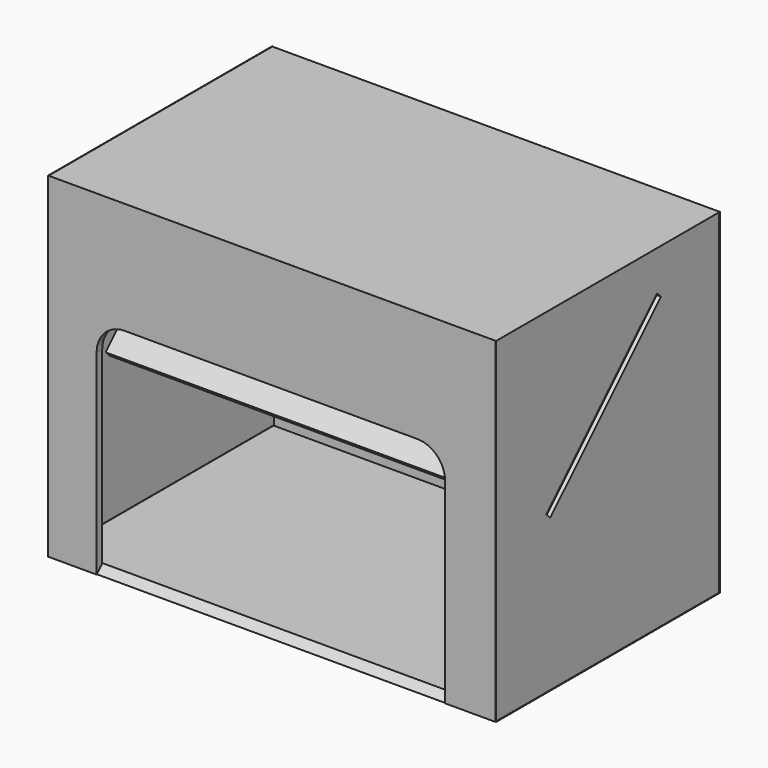
from build123d import *

# Parameters (mm, degrees)
F0_W           = 406.4
F0_H           = 254
F1_DEPTH       = 6.35
F2_SIZE        = 6.34999
F3_W           = 406.4
F3_H           = 304.8
F4_DEPTH       = 6.35
F5_SIZE        = 6.34999
F7_D           = 44.45
F7_CBORE_D     = 50.8
F7_CBORE_DEPTH = 3.175
F8_W           = 192.7503757179
F8_H           = 6.3895136118
F9_DEPTH       = 355.6
F10_ANGLE      = -45
F13_SIZE       = 2.54
F17_W          = 254
F17_H          = 304.8
F18_DEPTH      = 6.35
F20_SIZE       = 6.34999
F22_DEPTH      = 400.05
F24_DEPTH      = 3.175
F25_W          = 349.25
F25_H          = 127
F26_DEPTH      = 3.175
F29_DEPTH      = 25.4
F30_W          = 406.4
F30_H          = 304.8
F31_DEPTH      = 6.35
F32_SIZE       = 6.34999
F35_DEPTH      = 6.35
F39_W          = 406.4
F39_H          = 254
F40_DEPTH      = 6.35
F43_W          = 406.4
F43_H          = 254
F44_DEPTH      = 6.35
F46_SIZE       = 6.34999


# Not quite as in the source:
# - a fillet or chamfer is up to 0.001 mm smaller than in the source, because OpenCascade refuses the exact size


with BuildPart() as f1:
    # F0 (on Top) → F1 (new body)
    with BuildSketch(Plane.XY):
        with Locations((4.1009858251, 30.9985745514)):
            Rectangle(F0_W, F0_H)
    extrude(amount=F1_DEPTH)

    # F2 (size 6.35 in the source; OpenCascade refuses exactly that, so slightly less here)
    f2_edges = [f1.edges().sort_by_distance(p)[0] for p in [
        (-199.099014, 30.998575, 6.35),
        (4.100986, 157.998575, 6.35),
        (4.100986, -96.001425, 6.35),
        (207.300986, 30.998575, 6.35),
    ]]
    chamfer(f2_edges, length=F2_SIZE)


with BuildPart() as f4:
    # F3 (on Front) → F4 (new body)
    with BuildSketch(Plane.XZ):
        with Locations((84.3813158572, 276.6985837005)):
            Rectangle(F3_W, F3_H)
    extrude(amount=F4_DEPTH)

    # F5 (size 6.35 in the source; OpenCascade refuses exactly that, so slightly less here)
    f5_edges = [f4.edges().sort_by_distance(p)[0] for p in [
        (84.381316, -6.35, 124.298584),
        (287.581316, -6.35, 276.698584),
        (-118.818684, -6.35, 276.698584),
        (84.381316, -6.35, 429.098584),
    ]]
    chamfer(f5_edges, length=F5_SIZE)

    # F7 (through all)
    with Locations(Plane(origin=(0, 0, 0), x_dir=(-1, 0, 0), z_dir=(0, 1, 0))):
        with Locations((-84.3885657899, 327.5033756889)):
            CounterBoreHole(F7_D / 2, F7_CBORE_D / 2, F7_CBORE_DEPTH)


with BuildPart() as f9:
    # F8 (on Right) → F9 (new body)
    with BuildSketch(Plane.YZ):
        with Locations((-139.9461273104, 135.7569471002)):
            Rectangle(F8_W, F8_H)
    extrude(amount=F9_DEPTH)


with BuildPart() as f9_1:
    # F10: moved
    add(f9.part.rotate(Axis((177.8, -236.3213151693, 132.5621902943), (-1, 0, 0)), F10_ANGLE))


with BuildPart() as f9_2:
    # F11: moved
    add(f9_1.part.moved(Location((-101.6, 0, 0))))


with BuildPart() as f9_3:
    # F12: moved
    add(f9_2.part.moved(Location((0, 71.8420489686, -71.8420489686))))

    # F13
    f13_edges = [f9_3.edges().sort_by_distance(p)[0] for p in [
        (254, -96.331717, 128.86769),
        (254, -100.849786, 133.385759),
    ]]
    chamfer(f13_edges, length=F13_SIZE)


with BuildPart() as f4_1:
    # F14: moved
    add(f4.part.moved(Location((0, 152.4, -127))))


with BuildPart() as f1_1:
    # F15: moved
    add(f1.part.moved(Location((0, -5.08, -2.54))))


with BuildPart() as f4_2:
    # F16: moved
    add(f4_1.part.moved(Location((-80.01, 0, 0))))


with BuildPart() as f18:
    # F17 (on Right) → F18 (new body)
    with BuildSketch(Plane.YZ):
        with Locations((26.0427181125, 152.4)):
            Rectangle(F17_W, F17_H)
    extrude(amount=F18_DEPTH)


with BuildPart() as f18_1:
    # F19: moved
    add(f18.part.moved(Location((-199.39, 0, -2.54))))

    # F20 (size 6.35 in the source; OpenCascade refuses exactly that, so slightly less here)
    f20_edges = [f18_1.edges().sort_by_distance(p)[0] for p in [
        (-193.04, 26.042718, -2.54),
        (-193.04, -100.957282, 149.86),
        (-193.04, 153.042718, 149.86),
        (-193.04, 26.042718, 302.26),
    ]]
    chamfer(f20_edges, length=F20_SIZE)

    # F23 (on face) → F24 (cut)
    with BuildSketch(Plane.YZ.offset(-193.04)):
        Polygon((81.6913265085, 265.7688767814), (-44.0322591865, 140.0452910864), (-39.5421311259, 135.5551630259), (86.181454569, 261.2787487208), align=None)
    extrude(amount=-F24_DEPTH, mode=Mode.SUBTRACT)


with BuildPart() as f22:
    # F21 (on Right) → F22 (new body)
    with BuildSketch(Plane.YZ):
        Polygon((78.2378035879, 276.3127596282), (-47.4857821071, 150.5891739332), (-42.9956540465, 146.0990458727), (82.7279316484, 271.8226315677), align=None)
    extrude(amount=F22_DEPTH)

    # F25 (on face) → F26 (cut)
    with BuildSketch(Plane(origin=(0, -94.5473499596, 94.5473499596), x_dir=(1, 0, 0), z_dir=(0, 0.7071067812, -0.7071067812))):
        with Locations((200.02202293, -161.8170156378)):
            Rectangle(F25_W, F25_H)
    extrude(amount=-F26_DEPTH, mode=Mode.SUBTRACT)


with BuildPart() as f27_1:
    # F27: copy of F18
    add(f18_1.part)


with BuildPart() as f18_2:
    add(f18_1.part)

    # F23 (on face) → F29 (cut)
    with BuildSketch(Plane.YZ.offset(-193.04)):
        Polygon((81.6913265085, 265.7688767814), (-44.0322591865, 140.0452910864), (-39.5421311259, 135.5551630259), (86.181454569, 261.2787487208), align=None)
    extrude(amount=-F29_DEPTH, mode=Mode.SUBTRACT)


with BuildPart() as f31:
    # F30 (on Front) → F31 (new body)
    with BuildSketch(Plane.XZ):
        with Locations((6.1595166445, 152.4)):
            Rectangle(F30_W, F30_H)
    extrude(amount=F31_DEPTH)

    # F32 (size 6.35 in the source; OpenCascade refuses exactly that, so slightly less here)
    f32_edges = [f31.edges().sort_by_distance(p)[0] for p in [
        (209.359517, 0, 152.4),
        (6.159517, 0, 0),
        (-197.040483, 0, 152.4),
        (6.159517, 0, 304.8),
    ]]
    chamfer(f32_edges, length=F32_SIZE)


with BuildPart() as f31_1:
    # F33: moved
    add(f31.part.moved(Location((-2.54, -95.25, 0))))


with BuildPart() as f35_tool:
    # F34 (on face) → F35 (new body)
    with BuildSketch(Plane.XZ.offset(101.6)):
        with BuildLine():
            Line((-155.3397791949, 177.8), (-155.3397791949, 0))
            Line((-155.3397791949, 0), (161.1733883619, 0))
            Line((161.1733883619, 0), (161.1733883619, 177.8))
            ThreePointArc((161.1733883619, 177.8), (153.7339006041, 195.7605122421), (135.7733883619, 203.2))
            Line((135.7733883619, 203.2), (-129.9397791949, 203.2))
            ThreePointArc((-129.9397791949, 203.2), (-147.900291437, 195.7605122421), (-155.3397791949, 177.8))
        make_face()
    extrude(amount=-F35_DEPTH)


with BuildPart() as f9_4:
    add(f9_3.part)

    # F35: cut by f35_tool
    add(f35_tool.part, mode=Mode.SUBTRACT)


with BuildPart() as f31_2:
    add(f31_1.part)

    # F35: cut by f35_tool
    add(f35_tool.part, mode=Mode.SUBTRACT)


with BuildPart() as f22_1:
    # F37: moved
    add(f22.part.moved(Location((-196.85, 3.556, -11.176))))


with BuildPart() as f31_3:
    # F38: moved
    add(f31_2.part.moved(Location((0, 0, -2.54))))


with BuildPart() as f40:
    # F39 (on Top) → F40 (new body)
    with BuildSketch(Plane.XY):
        with Locations((4.5869623899, 24.6496979594)):
            Rectangle(F39_W, F39_H)
    extrude(amount=F40_DEPTH)


with BuildPart() as f40_1:
    # F41: moved
    add(f40.part.moved(Location((0, 1.27, 295.91))))


with BuildPart() as f44:
    # F43 (on Top) → F44 (new body)
    with BuildSketch(Plane.XY):
        with Locations((4.2246704578, 26.4611725211)):
            Rectangle(F43_W, F43_H)
    extrude(amount=F44_DEPTH)


with BuildPart() as f44_1:
    # F45: moved
    add(f44.part.moved(Location((0, -1.016, 295.91))))

    # F46 (size 6.35 in the source; OpenCascade refuses exactly that, so slightly less here)
    f46_edges = [f44_1.edges().sort_by_distance(p)[0] for p in [
        (4.22467, -101.554827, 295.91),
        (-198.97533, 25.445173, 295.91),
        (4.22467, 152.445173, 295.91),
        (207.42467, 25.445173, 295.91),
    ]]
    chamfer(f46_edges, length=F46_SIZE)


with BuildPart() as f47_1:
    # F47: instance of F18
    add(f18_2.part.mirror(Plane.YZ))


with BuildPart() as f47_1_1:
    # F48: moved
    add(f47_1.part)


with BuildPart() as f47_1_2:
    # F49: moved
    add(f47_1_1.part.moved(Location((7.62, 0, 0))))


solid = Compound([f1_1.part, f4_2.part, f18_2.part, f22_1.part, f31_3.part, f44_1.part, f47_1_2.part])
